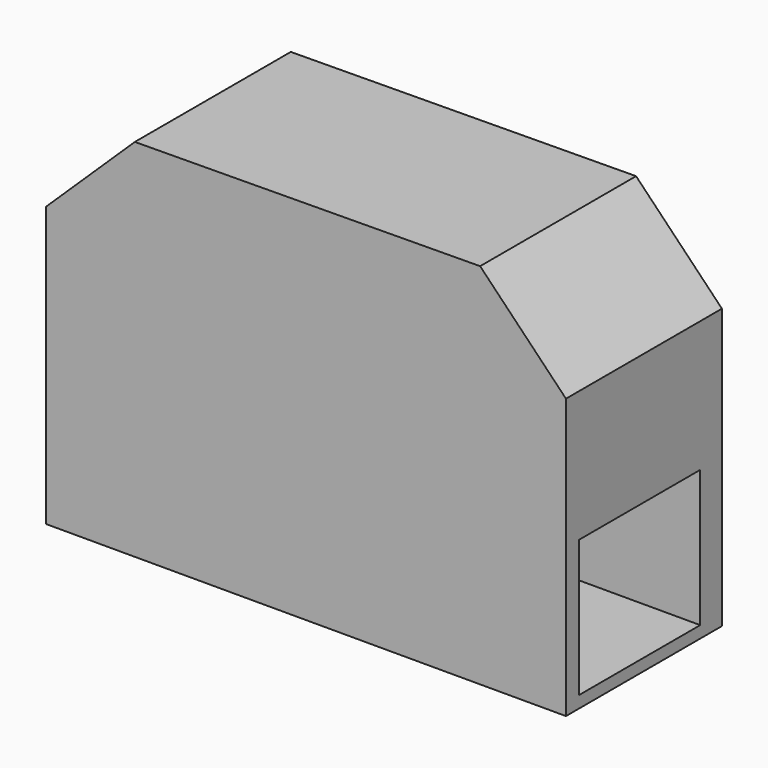
from build123d import *

# Parameters (mm, degrees)
F0_W     = 2032
F0_H     = 508
F1_DEPTH = 762
F2_W     = 591.2553668022
F2_H     = 534.2325568199
F3_DEPTH = 2032


with BuildPart() as f1:
    # F0 (on Front) → F1 (new body)
    with BuildSketch(Plane.XZ):
        Polygon((1016, 0), (0, 0), (-1016, 0), (-1016, -76.2), (1016, -76.2), align=None)
        Polygon((-1016, 0), (0, 0), (1016, 0), (1016, 508), (-1016, 508), align=None)
        with Locations((0, 762)):
            Rectangle(F0_W, F0_H)
        Polygon((-669.1186458851, 1351.5236000156), (-1016, 1016), (1016, 1016), (680.4763999844, 1362.8813541149), align=None)
    extrude(amount=F1_DEPTH)

    # F2 (on face) → F3 (cut)
    with BuildSketch(Plane(origin=(-1016, 0, 0), x_dir=(0, -1, 0), z_dir=(-1, 0, 0))):
        with Locations((401.707559824, 237.3584806919)):
            Rectangle(F2_W, F2_H)
    extrude(amount=-F3_DEPTH, mode=Mode.SUBTRACT)


solid = f1.part
